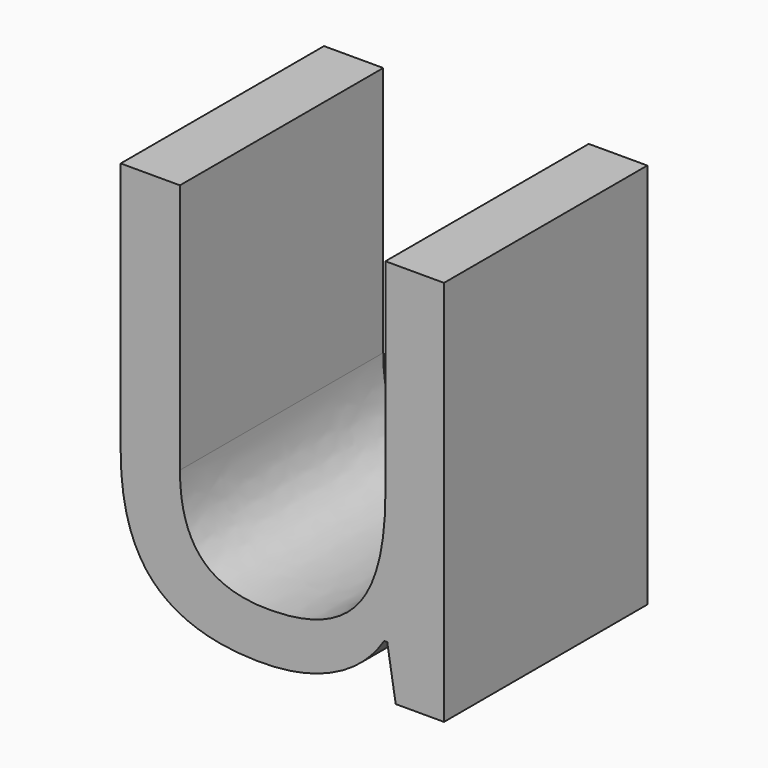
from build123d import *

# Parameters (mm, degrees)
F0_TEXT_SIZE = 36.0932113836
F1_DEPTH     = 12.7


# Not quite as in the source:
# - Text() gives the source's letters only with a copy of the font that has no kerning and outlines rounded to 1/6400 em; it was checked with that copy


with BuildPart() as f1:
    # F0 (on Front) → F1 (new body)
    with BuildSketch(Plane.XZ):
        with Locations((-59.3705587089, 3.3983110916)):
            Text('u', F0_TEXT_SIZE, font='Open Sans', text_align=(TextAlign.LEFT, TextAlign.BOTTOM))
    extrude(amount=F1_DEPTH)


solid = f1.part
